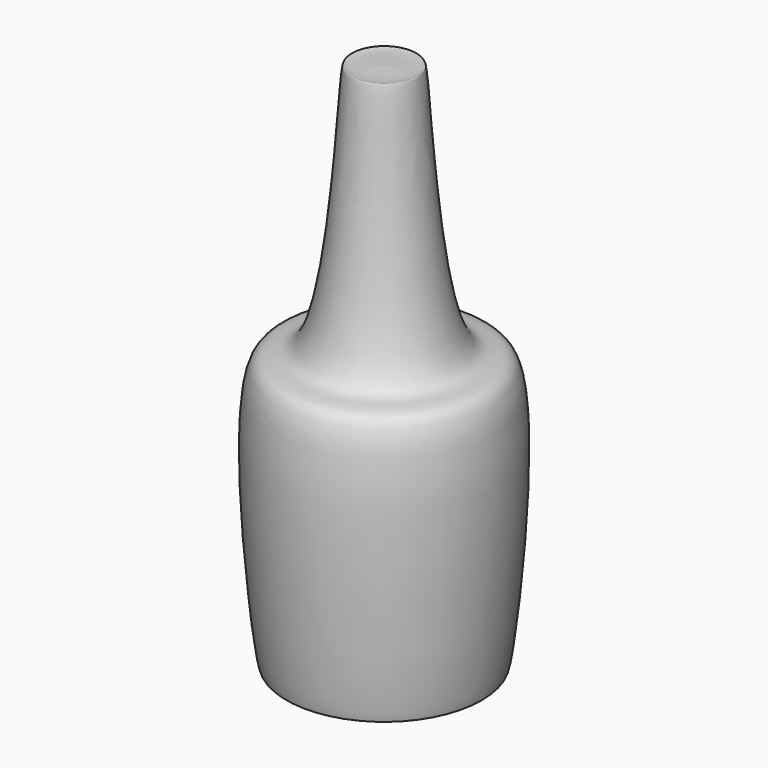
from build123d import *


# Not quite as in the source:
# - a feature of the source that left no trace in its solid (it failed there, or was rolled back) is left out


with BuildPart() as f5:
    # F4 (on Front) → F5 (revolve)
    with BuildSketch(Plane.XZ):
        with BuildLine():
            Line((-190.4045946752, 108.5054529886), (-190.4045946752, -141.4945470114))
            Line((-190.4045946752, -141.4945470114), (-144.424073361, -141.4945470114))
            Line((-144.424073361, -141.4945470114), (-144.1295946752, -141.4945470114))
            add(Edge.make_bspline(
                [(-190.4045946752, 108.5054529886), (-183.9120433877, 108.1774164313), (-176.0642613208, 107.7805812971), (-173.2680945383, 111.2709340537), (-169.6801899691, -28.2385328746), (-126.3264217306, 4.771776778), (-141.8682028974, -138.2167803471), (-144.1295946752, -141.4945470114)],
                knots=[0, 0, 0, 0, 0.1215749653, 0.1472155017, 0.4916045773, 0.6276587556, 0.9827770812, 0.9827770812, 0.9827770812, 0.9827770812], degree=3))
        make_face()
    revolve(axis=Axis((-190.4045946752, 0, -16.4945470114), (0, 0, 1)))


solid = f5.part
